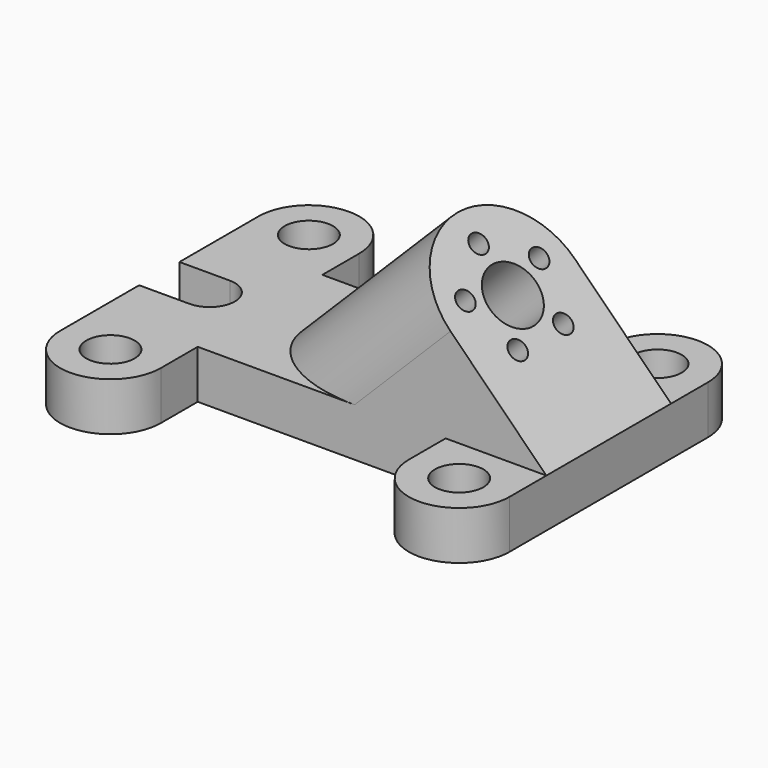
from build123d import *

# Parameters (mm, degrees)
F0_R     = 6.25
F1_DEPTH = 12.5
F3_R     = 2.5
F3_R_2   = 7.5
F4_REACH = 159.0869091096


with BuildPart() as f1:
    # F0 (on Top) → F1 (new body)
    with BuildSketch(Plane.XY):
        with BuildLine():
            Line((0, 32), (0, 6.5))
            Line((0, 6.5), (13, 6.5))
            ThreePointArc((13, 6.5), (19.5, 0), (13, -6.5))
            Line((13, -6.5), (0, -6.5))
            Line((0, -6.5), (0, -32))
            ThreePointArc((0, -32), (13, -45), (26, -32))
            Line((26, -32), (26, -20.1084308683))
            Line((26, -20.1084308683), (90, -20.1084308683))
            Line((90, -20.1084308683), (90, -32))
            ThreePointArc((90, -32), (103, -45), (116, -32))
            Line((116, -32), (116, 32))
            ThreePointArc((116, 32), (103, 45), (90, 32))
            Line((90, 32), (90, 20.1084308683))
            Line((90, 20.1084308683), (26, 20.1084308683))
            Line((26, 20.1084308683), (26, 32))
            ThreePointArc((26, 32), (13, 45), (0, 32))
        make_face()
        with Locations((13, -32)):
            Circle(F0_R, mode=Mode.SUBTRACT)
        with Locations((103, -32)):
            Circle(F0_R, mode=Mode.SUBTRACT)
        with Locations((13, 32)):
            Circle(F0_R, mode=Mode.SUBTRACT)
        with Locations((103, 32)):
            Circle(F0_R, mode=Mode.SUBTRACT)
    extrude(amount=F1_DEPTH)

    f4_end = f1.faces().sort_by_distance((59.8447932422, 0, 0))[0]
    # F3 (on face) → F4 (join, up to a face of the model that its end follows)
    with BuildSketch(Plane(origin=(64.25, 0, 64.25), x_dir=(0, -1, 0), z_dir=(-0.7071067812, 0, -0.7071067812))):
        with BuildLine():
            Line((-20.1084308683, -73.1855518528), (20.1084308683, -73.1855518528))
            Line((20.1084308683, -73.1855518528), (20.1084308683, -38.1855518528))
            ThreePointArc((20.1084308683, -38.1855518528), (0, -18.0771209845), (-20.1084308683, -38.1855518528))
            Line((-20.1084308683, -38.1855518528), (-20.1084308683, -73.1855518528))
        make_face()
        with Locations((-7.3473156537, -48.2982642825)):
            Circle(F3_R, mode=Mode.SUBTRACT)
        with Locations((7.3473156537, -48.2982642825)):
            Circle(F3_R, mode=Mode.SUBTRACT)
        with Locations((-11.8882064537, -34.3228394231)):
            Circle(F3_R, mode=Mode.SUBTRACT)
        with Locations((0, -38.1855518528)):
            Circle(F3_R_2, mode=Mode.SUBTRACT)
        with Locations((11.8882064537, -34.3228394231)):
            Circle(F3_R, mode=Mode.SUBTRACT)
        with Locations((0, -25.6855518528)):
            Circle(F3_R, mode=Mode.SUBTRACT)
    f4_long = extrude(amount=F4_REACH, mode=Mode.PRIVATE)
    add(split(f4_long, bisect_by=f4_end, keep=Keep.BOTTOM, mode=Mode.PRIVATE))


solid = f1.part
